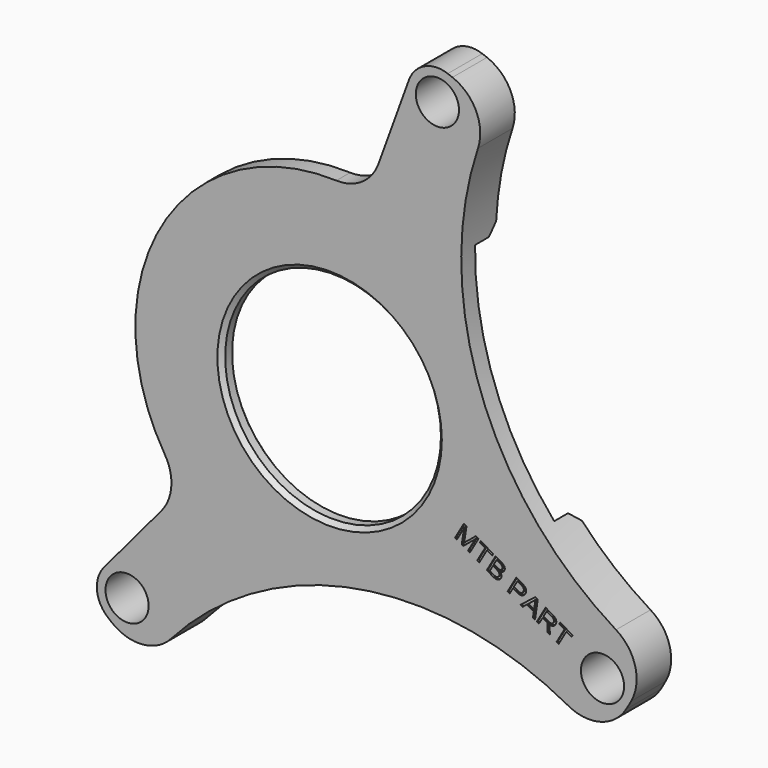
from build123d import *

# Parameters (mm, degrees)
F0_R         = 2.5
F0_R_2       = 12.5
F1_DEPTH     = 5
F2_R         = 25
F3_DEPTH     = 3
F4_SIZE      = 1
F5_SIZE      = 0.5
F6_TEXT_SIZE = 2.9399154774
F7_DEPTH     = 0.2


# Not quite as in the source:
# - Text() gives the source's letters only with a copy of the font that has no kerning and outlines rounded to 1/6400 em; it was checked with that copy


with BuildPart() as f1:
    # F0 (on Front) → F1 (new body)
    with BuildSketch(Plane.XZ):
        with BuildLine():
            ThreePointArc((-26.1429033045, -25.7108655399), (-26.9484291969, -28.2656672735), (-25.7115043875, -30.6417777248))
            ThreePointArc((-25.7115043875, -30.6417777248), (-25.4867966173, -30.8289344316), (-25.2607265585, -31.0144433085))
            ThreePointArc((-25.2607265585, -31.0144433085), (-21.6944353053, -32.1209062959), (-18.3560794496, -30.4481618967))
            ThreePointArc((-18.3560794496, -30.4481618967), (3.2350360563, -18.3468011719), (27.6629571012, -22.3337641266))
            ThreePointArc((27.6629571012, -22.3337641266), (31.3720977436, -22.7638447467), (34.3448826883, -20.5043661967))
            ThreePointArc((34.3448826883, -20.5043661967), (34.6410161514, -20), (34.929743359, -19.4913577997))
            ThreePointArc((34.929743359, -19.4913577997), (35.4001167103, -15.7871112426), (33.1730856464, -12.7899415302))
            ThreePointArc((33.1730856464, -12.7899415302), (17.5063139212, 6.371777179), (17.1908419763, 31.1209120656))
            ThreePointArc((17.1908419763, 31.1209120656), (16.9703031921, 34.8483852431), (14.2289325102, 37.383652572))
            ThreePointArc((14.2289325102, 37.383652572), (13.9552420807, 37.4866805475), (13.680805733, 37.5877048314))
            ThreePointArc((13.680805733, 37.5877048314), (11.0045713153, 37.4708579133), (9.1948110586, 35.4958511603))
            Line((9.1948110586, 35.4958511603), (5.6560632757, 25.7732215336))
            ThreePointArc((5.6560632757, 25.7732215336), (3.753725768, 23.3382430411), (0.7834910496, 22.4863545684))
            ThreePointArc((0.7834910496, 22.4863545684), (-19.4855715851, 11.25), (-19.0820087699, -11.9217004368))
            ThreePointArc((-19.0820087699, -11.9217004368), (-18.3346484693, -14.9199433945), (-19.4922329476, -17.784905249))
            Line((-19.4922329476, -17.784905249), (-26.1429033045, -25.7108655399))
        make_face()
        with Locations((-23.4617477536, -27.9606221738)):
            Circle(F0_R, mode=Mode.SUBTRACT)
        Circle(F0_R_2, mode=Mode.SUBTRACT)
        with Locations((31.6099272381, -18.25)):
            Circle(F0_R, mode=Mode.SUBTRACT)
        with Locations((12.4837352314, 34.2987806587)):
            Circle(F0_R, mode=Mode.SUBTRACT)
    extrude(amount=F1_DEPTH)

    # F2 (on face) → F3 (cut)
    with BuildSketch(Plane(origin=(0, 0, 0), x_dir=(-1, 0, 0), z_dir=(0, 1, 0))):
        Circle(F2_R)
    extrude(amount=-F3_DEPTH, mode=Mode.SUBTRACT)

    # F4
    f4_edges = [f1.edges().sort_by_distance(p)[0] for p in [
        (10.378709, 0, 22.743843),
        (21.650635, 0, -12.5),
        (-14.507391, 0, -20.360147),
    ]]
    chamfer(f4_edges, length=F4_SIZE)

    # F5
    f5_edges = [f1.edges().sort_by_distance(p)[0] for p in [
        (-12.5, -3, 0),
        (12.5, -4, 0),
        (-12.5, -5, 0),
    ]]
    chamfer(f5_edges, length=F5_SIZE)

    # F6 (on face) → F7 (cut)
    with BuildSketch(Plane.XZ.offset(5)):
        with Locations(Location((14.3233851977, -9.3358156282), (0, 0, -30))):
            Text('MTB PART', F6_TEXT_SIZE, font='Arimo', text_align=(TextAlign.LEFT, TextAlign.BOTTOM))
    extrude(amount=-F7_DEPTH, mode=Mode.SUBTRACT)


solid = f1.part
